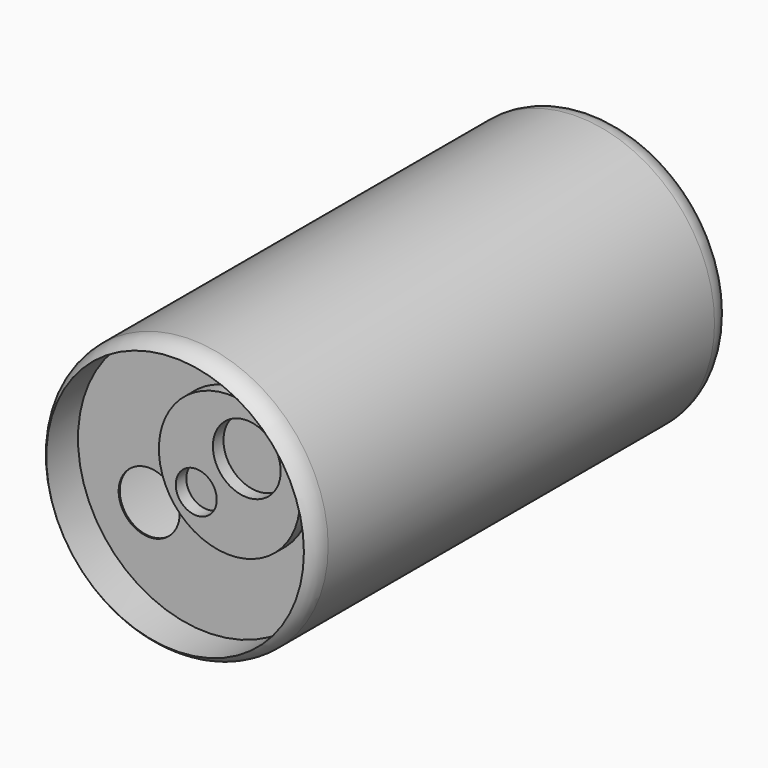
from build123d import *

# Parameters (mm, degrees)
F0_R      = 26.403137542
F1_DEPTH  = 101.6
F2_R      = 24.74377178
F3_DEPTH  = 7.62
F5_R      = 13.5480527637
F6_DEPTH  = 2.54
F7_R      = 6.5142551247
F8_DEPTH  = 2.54
F9_R      = 3.938583422
F10_DEPTH = 2.54
F11_T     = -0.254
F12_R     = 21.153794525
F13_DEPTH = 0.254
F14_R     = 5.8596108627
F15_DEPTH = 25.4


# Not quite as in the source:
# - a fillet or chamfer that OpenCascade refuses, or shapes differently, is made with other operations: its cross-section is extruded or revolved along the edge and cut away or added
# - a shell that OpenCascade refuses in one call is made with other operations: the cavity is built on its own and cut out


with BuildPart() as f1:
    # F0 (on Front) → F1 (new body)
    with BuildSketch(Plane.XZ):
        Circle(F0_R)
    extrude(amount=F1_DEPTH)

    # F2 (on face) → F3 (cut)
    with BuildSketch(Plane.XZ.offset(101.6)):
        Circle(F2_R)
    extrude(amount=-F3_DEPTH, mode=Mode.SUBTRACT)

    # F4: fillet of radius 5.08 on 2 edges, made by hand

    # F4_s1 → F4_t2 (revolve, cut)
    with BuildSketch(Plane.XY):
        with BuildLine():
            ThreePointArc((26.403137542, -97.8442495544), (25.9698149533, -99.8972446921), (24.74377178, -101.6))
            Line((24.74377178, -101.6), (24.8121844648, -101.6751150089))
            ThreePointArc((24.8121844648, -101.6751150089), (25.573454661, -101.7016), (26.403137542, -101.7016))
            Line((26.403137542, -101.7016), (26.504737542, -101.6))
            Line((26.504737542, -101.6), (26.504737542, -97.8442495544))
            Line((26.504737542, -97.8442495544), (26.403137542, -97.8442495544))
        make_face()
    revolve(axis=Axis((0, -101.6, 0), (0, -1, 0)), mode=Mode.SUBTRACT)

    # F4_s3 → F4_t4 (revolve, cut)
    with BuildSketch(Plane.XY):
        with BuildLine():
            ThreePointArc((26.403137542, -5.08), (24.9152399905, -1.4878975516), (21.323137542, 0))
            Line((21.323137542, 0), (21.323137542, 0.1016))
            Line((21.323137542, 0.1016), (26.504737542, 0.1016))
            Line((26.504737542, 0.1016), (26.504737542, -5.08))
            Line((26.504737542, -5.08), (26.403137542, -5.08))
        make_face()
    revolve(axis=Axis((0, 0, 0), (0, -1, 0)), mode=Mode.SUBTRACT)

    # F5 (on face) → F6 (join)
    with BuildSketch(Plane.XZ.offset(93.98)):
        with Locations((6.3713835552, 5.0060865469)):
            Circle(F5_R)
    extrude(amount=F6_DEPTH)

    # F7 (on face) → F8 (cut)
    with BuildSketch(Plane.XZ.offset(96.52)):
        with Locations((9.7087752074, 8.7985796854)):
            Circle(F7_R)
    extrude(amount=-F8_DEPTH, mode=Mode.SUBTRACT)

    # F9 (on face) → F10 (cut)
    with BuildSketch(Plane.XZ.offset(96.52)):
        Circle(F9_R)
    extrude(amount=-F10_DEPTH, mode=Mode.SUBTRACT)

    # F11: a shell. OpenCascade refuses it in one call, so the cavity is built on its own and cut out:
    # the body offset inwards by the wall thickness, plus a prism from it out through each open face.
    f11_core = offset(f1.part, amount=F11_T, kind=Kind.INTERSECTION, mode=Mode.PRIVATE)
    f11_exits = [f11_core.faces().sort_by_distance(p)[0] for p in [
        (0, -0.254, 0),
    ]]
    add(f11_core, mode=Mode.SUBTRACT)
    extrude(f11_exits, amount=-F11_T, mode=Mode.SUBTRACT)

    # F14 (on face) → F15 (cut)
    with BuildSketch(Plane.XZ.offset(93.98)):
        with Locations((-11.0740670934, -6.3713807613)):
            Circle(F14_R)
    extrude(amount=-F15_DEPTH, mode=Mode.SUBTRACT)


with BuildPart() as f13:
    # F12 (on Front) → F13 (new body)
    with BuildSketch(Plane.XZ):
        Circle(F12_R)
    extrude(amount=F13_DEPTH)


solid = Compound([f1.part, f13.part])
